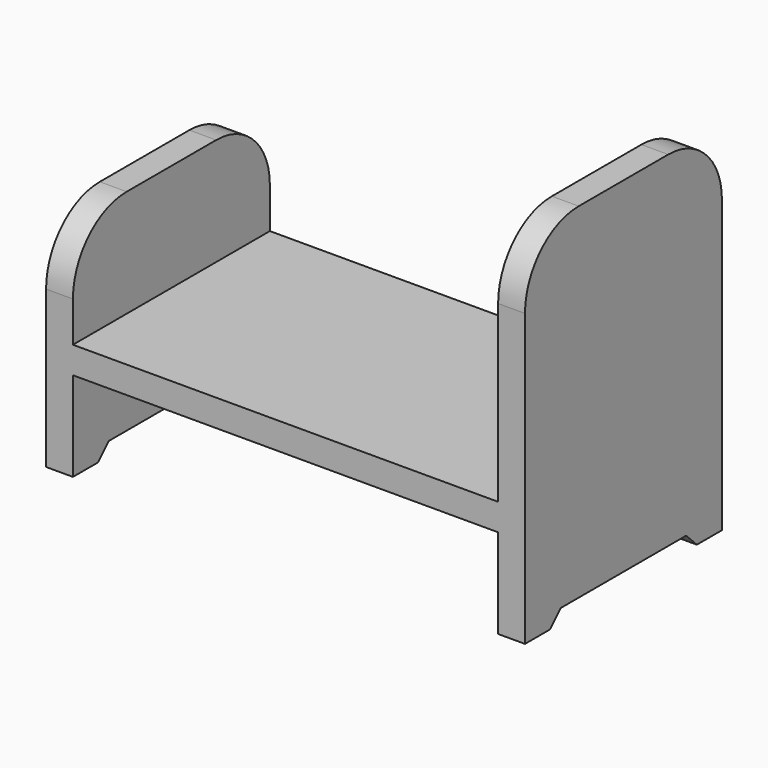
from build123d import *

# Parameters (mm, degrees)
F1_DEPTH     = 55
F2_R         = 15
F4_DEPTH     = 107.001
F6_DEPTH     = 2
F7_TEXT_SIZE = 9.7410362897
F8_DEPTH     = 1


# Not quite as in the source:
# - Text() gives the source's letters only with a copy of the font that has no kerning and outlines rounded to 1/6400 em; it was checked with that copy


with BuildPart() as f1:
    # F0 (on Front) → F1 (new body)
    with BuildSketch(Plane.XZ):
        Polygon((0, 50), (0, 0), (6, 0), (6, 20), (101, 20), (101, 0), (107, 0), (107, 80), (101, 80), (101, 26), (6, 26), (6, 50), align=None)
    extrude(amount=F1_DEPTH)

    # F2
    f2_edges = [f1.edges().sort_by_distance(p)[0] for p in [
        (104, -55, 80),
        (104, 0, 80),
        (3, -55, 50),
        (3, 0, 50),
    ]]
    fillet(f2_edges, radius=F2_R)

    # F3 (on face) → F4 (cut, through all)
    with BuildSketch(Plane(origin=(0, 0, 0), x_dir=(0, -1, 0), z_dir=(-1, 0, 0))):
        Polygon((10, 3), (7, 0), (48, 0), (45, 3), align=None)
    extrude(amount=-F4_DEPTH, mode=Mode.SUBTRACT)

    # F5 (on face) → F6 (cut)
    with BuildSketch(Plane(origin=(101, 0, 0), x_dir=(0, -1, 0), z_dir=(-1, 0, 0))):
        Polygon((33.4930710421, 71.6276506646), (33.3276427515, 71.0721378586), (30.6165331563, 63.9000498928), (22.8960190098, 66.1991714324), (28.5177540672, 61.5143916883), (24.0057140536, 58.936095349), (28.6466707202, 58.936095349), (25.4237849961, 52.2095398324), (30.2931282559, 57.3891077535), (31.9506276313, 52.2095398324), (33.4930710421, 57.3891077535), (39.0298717548, 53.7794720706), (34.5767786164, 58.936095349), (39.0298717548, 60.3611175145), (35.9071828227, 61.2910350367), (39.0298717548, 63.9000498928), (34.5767786164, 63.3192125898), align=None)
        Polygon((15.8258866344, 74.4129480422), (15.0000458824, 72.2364628476), (12.7359506074, 72.2369402034), (14.5856735493, 70.9472963181), (13.9545143851, 69.4951678786), (15.6906694975, 70.0264648313), (17.4402487104, 68.7372983018), (16.6115009843, 70.118545532), (18.4992043083, 71.4077120615), (16.7398117626, 71.6276506646), align=None)
        Polygon((43.8618634114, 73.3462407134), (42.3414251726, 71.5834678093), (40.2140348153, 72.3582825674), (41.5111216278, 70.5137712193), (40.4213688416, 69.365085988), (42.2345352492, 69.2705417936), (43.4376810039, 67.4607301856), (43.1313272568, 69.0421264314), (45.3461090618, 69.6079141448), (43.7680443021, 70.4163365177), align=None)
        Polygon((44.179189826, 52.4783079998), (43.353349074, 50.3018228053), (41.089253799, 50.3023001611), (42.938976741, 49.0126562758), (42.3078175768, 47.5605278362), (44.0439726891, 48.091824789), (45.7935519021, 46.8026582595), (44.964804176, 48.1839054897), (46.8525074999, 49.4730720192), (45.0931149543, 49.6930106223), align=None)
        Polygon((23.6659891443, 50.0885977825), (22.8401483923, 47.912112588), (20.5760531173, 47.9125899437), (22.4257760592, 46.6229460585), (21.794616895, 45.1708176189), (23.5307720074, 45.7021145717), (25.2803512203, 44.4129480422), (24.4516034942, 45.7941952724), (26.3393068182, 47.0833618019), (24.5799142725, 47.303300405), align=None)
        Polygon((10.4159199481, 60.4334293783), (9.5900791961, 58.2569441838), (7.3259839211, 58.2574215396), (9.175706863, 56.9677776543), (8.5445476988, 55.5156492148), (10.2807028112, 56.0469461675), (12.0302820242, 54.757779638), (11.201534298, 56.1390268682), (13.089237622, 57.4281933977), (11.3298450764, 57.6481320008), align=None)
    extrude(amount=-F6_DEPTH, mode=Mode.SUBTRACT)

    # F7 (on face) → F8 (cut)
    with BuildSketch(Plane(origin=(0, 0, 20), x_dir=(1, 0, 0), z_dir=(0, 0, -1))):
        with Locations((18.4270006355, 22.8450255458)):
            Text('Beth 18/2/2017', F7_TEXT_SIZE, font='Open Sans', text_align=(TextAlign.LEFT, TextAlign.BOTTOM))
    extrude(amount=-F8_DEPTH, mode=Mode.SUBTRACT)


solid = f1.part
